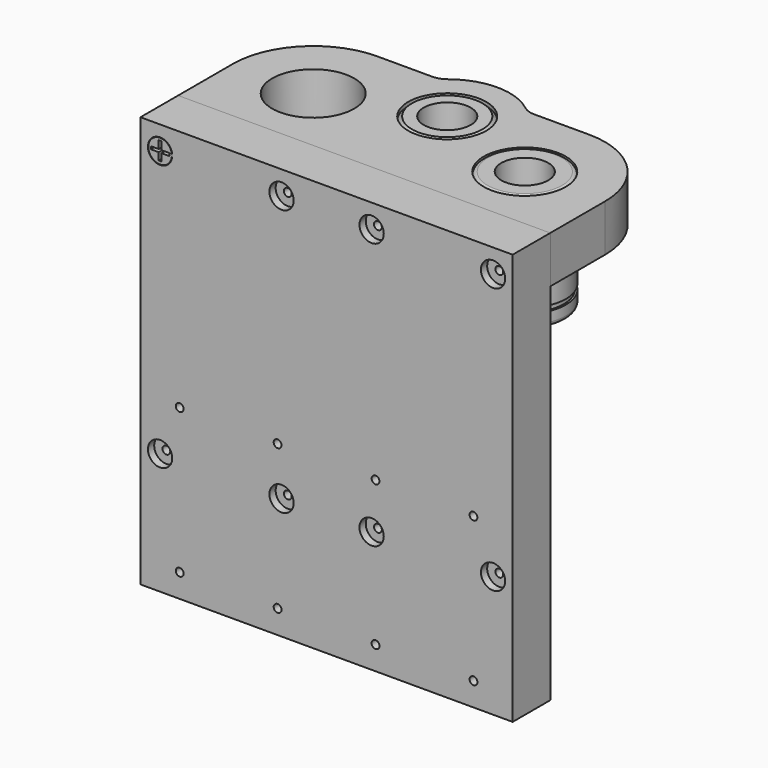
from build123d import *

# Parameters (mm, degrees)
F0_W      = 95
F0_H      = 80
F1_DEPTH  = 12
F2_R      = 10.475
F3_DEPTH  = 12
F4_R      = 9.975
F5_DEPTH  = 25
F6_R      = 10.5
F6_R_2    = 6
F7_DEPTH  = 30
F9_START  = -3.5
F8_R      = 13.9480454754
F8_R_2    = 10
F9_DEPTH  = 1.3
F11_START = -3.5
F10_R     = 14.6955703702
F10_R_2   = 10
F11_DEPTH = 1.3
F12_R     = 1
F13_R     = 1
F14_DEPTH = 25
F15_R     = 3.1
F16_DEPTH = 2
F17_R     = 3
F18_DEPTH = 2
F19_R     = 0.95
F20_DEPTH = 23
F22_DEPTH = 1.5
F23_W     = 95
F23_H     = 25
F24_DEPTH = 12
F25_R     = 1
F26_DEPTH = 25
F27_R     = 3.1
F28_DEPTH = 2
F29_R     = 10
F29_R_2   = 6
F30_DEPTH = 25
F31_SIZE  = 1
F32_R     = 5


with BuildPart() as f1:
    # F0 (on Front) → F1 (new body)
    with BuildSketch(Plane.XZ):
        with Locations((0, 40)):
            Rectangle(F0_W, F0_H)
    extrude(amount=-F1_DEPTH)


with BuildPart() as f3:
    # F2 (on face) → F3 (new body)
    with BuildSketch(Plane.XY.offset(80)):
        with BuildLine():
            Line((-47.5, 12), (47.5, 12))
            Line((47.5, 12), (47.5, 29.5))
            ThreePointArc((47.5, 29.5), (41.4956890143, 43.9956890143), (27, 50))
            Line((27, 50), (11.1242977306, 50))
            ThreePointArc((11.1242977306, 50), (14.7307291688, 44.7454477946), (16, 38.5))
            ThreePointArc((16, 38.5), (-6.2454477946, 23.7692708312), (-11.1242977306, 50))
            Line((-11.1242977306, 50), (-27, 50))
            ThreePointArc((-27, 50), (-41.4956890143, 43.9956890143), (-47.5, 29.5))
            Line((-47.5, 29.5), (-47.5, 12))
        make_face()
        with Locations((-27, 29.5)):
            Circle(F2_R, mode=Mode.SUBTRACT)
        with Locations((27, 29.5)):
            Circle(F2_R, mode=Mode.SUBTRACT)
        with BuildLine():
            ThreePointArc((16, 38.5), (14.7307291688, 44.7454477946), (11.1242977306, 50))
            Line((11.1242977306, 50), (-11.1242977306, 50))
            ThreePointArc((-11.1242977306, 50), (-6.2454477946, 23.7692708312), (16, 38.5))
        make_face()
        with BuildLine():
            Line((-11.1242977306, 50), (11.1242977306, 50))
            ThreePointArc((11.1242977306, 50), (0, 54.5), (-11.1242977306, 50))
        make_face()
    extrude(amount=-F3_DEPTH)

    # F4 (on face) → F5 (cut)
    with BuildSketch(Plane.XY.offset(80)):
        with Locations((0, 38.5)):
            Circle(F4_R)
    extrude(amount=-F5_DEPTH, mode=Mode.SUBTRACT)


with BuildPart() as f7:
    # F6 (on face) → F7 (new body)
    with BuildSketch(Plane.XY.offset(80)):
        with Locations((27, 29.5)):
            Circle(F6_R)
        with Locations((27, 29.5)):
            Circle(F6_R_2, mode=Mode.SUBTRACT)
    extrude(amount=-F7_DEPTH)

    # F8 (on face) → F9 (cut)
    with BuildSketch(Plane.XY.offset(80).offset(F9_START)):
        with Locations((27, 29.5)):
            Circle(F8_R)
        with Locations((27, 29.5)):
            Circle(F8_R_2, mode=Mode.SUBTRACT)
    extrude(amount=-F9_DEPTH, mode=Mode.SUBTRACT)

    # F10 (on face) → F11 (cut)
    with BuildSketch(Plane(origin=(0, 0, 50), x_dir=(1, 0, 0), z_dir=(0, 0, -1)).offset(F11_START)):
        with Locations((27, -29.5)):
            Circle(F10_R)
        with Locations((27, -29.5)):
            Circle(F10_R_2, mode=Mode.SUBTRACT)
    extrude(amount=-F11_DEPTH, mode=Mode.SUBTRACT)

    # F12
    f12_edges = [f7.edges().sort_by_distance(p)[0] for p in [
        (16.5, 29.5, 80),
        (16.5, 29.5, 50),
    ]]
    fillet(f12_edges, radius=F12_R)


with BuildPart() as f14_tool:
    # F13 (on face) → F14 (new body)
    with BuildSketch(Plane.XZ):
        with Locations((-42.5, 74)):
            Circle(F13_R)
        with Locations((-11.5, 74)):
            Circle(F13_R)
        with Locations((11.5, 74)):
            Circle(F13_R)
        with Locations((42.5, 74)):
            Circle(F13_R)
        with Locations((-42.5, 6)):
            Circle(F13_R)
        with Locations((-11.5, 6)):
            Circle(F13_R)
        with Locations((11.5, 6)):
            Circle(F13_R)
        with Locations((42.5, 6)):
            Circle(F13_R)
    extrude(amount=-F14_DEPTH)


with BuildPart() as f1_1:
    add(f1.part)

    # F14: cut by f14_tool
    add(f14_tool.part, mode=Mode.SUBTRACT)

    # F15 (on face) → F16 (cut)
    with BuildSketch(Plane.XZ):
        with Locations((-42.5, 74)):
            Circle(F15_R)
        with Locations((-11.5, 74)):
            Circle(F15_R)
        with Locations((11.5, 74)):
            Circle(F15_R)
        with Locations((42.5, 74)):
            Circle(F15_R)
        with Locations((-42.5, 6)):
            Circle(F15_R)
        with Locations((-11.5, 6)):
            Circle(F15_R)
        with Locations((11.5, 6)):
            Circle(F15_R)
        with Locations((42.5, 6)):
            Circle(F15_R)
    extrude(amount=-F16_DEPTH, mode=Mode.SUBTRACT)

    # F23 (on face) → F24 (join)
    with BuildSketch(Plane.XZ):
        with Locations((0, -12.5)):
            Rectangle(F23_W, F23_H)
    extrude(amount=-F24_DEPTH)

    # F25 (on face) → F26 (cut)
    with BuildSketch(Plane(origin=(0, 12, 0), x_dir=(-1, 0, 0), z_dir=(0, 1, 0))):
        with Locations((-37.5, -19)):
            Circle(F25_R)
        with Locations((-37.5, 18)):
            Circle(F25_R)
        with Locations((-12.5, -19)):
            Circle(F25_R)
        with Locations((-12.5, 18)):
            Circle(F25_R)
        with Locations((12.5, -19)):
            Circle(F25_R)
        with Locations((12.5, 18)):
            Circle(F25_R)
        with Locations((37.5, -19)):
            Circle(F25_R)
        with Locations((37.5, 18)):
            Circle(F25_R)
    extrude(amount=-F26_DEPTH, mode=Mode.SUBTRACT)

    # F27 (on face) → F28 (cut)
    with BuildSketch(Plane(origin=(0, 12, 0), x_dir=(-1, 0, 0), z_dir=(0, 1, 0))):
        with Locations((-37.5, 18)):
            Circle(F27_R)
        with Locations((-37.5, -19)):
            Circle(F27_R)
        with Locations((-12.5, 18)):
            Circle(F27_R)
        with Locations((-12.5, -19)):
            Circle(F27_R)
        with Locations((12.5, 18)):
            Circle(F27_R)
        with Locations((12.5, -19)):
            Circle(F27_R)
        with Locations((37.5, 18)):
            Circle(F27_R)
        with Locations((37.5, -19)):
            Circle(F27_R)
    extrude(amount=-F28_DEPTH, mode=Mode.SUBTRACT)


with BuildPart() as f3_1:
    add(f3.part)

    # F14: cut by f14_tool
    add(f14_tool.part, mode=Mode.SUBTRACT)

    # F32
    f32_edges = [f3_1.edges().sort_by_distance(p)[0] for p in [
        (11.124298, 50, 74),
        (-11.124298, 50, 74),
    ]]
    fillet(f32_edges, radius=F32_R)


with BuildPart() as f18:
    # F17 (on face) → F18 (new body)
    with BuildSketch(Plane.XZ):
        with Locations((-42.5, 74)):
            Circle(F17_R)
    extrude(amount=-F18_DEPTH)

    # F19 (on face) → F20 (join)
    with BuildSketch(Plane(origin=(0, 2, 0), x_dir=(-1, 0, 0), z_dir=(0, 1, 0))):
        with Locations((42.5, 74)):
            Circle(F19_R)
    extrude(amount=F20_DEPTH)

    # F21 (on face) → F22 (cut)
    with BuildSketch(Plane.XZ):
        Polygon((-40.15, 73.65), (-40.15, 74.35), (-42.15, 74.35), (-42.15, 76.35), (-42.85, 76.35), (-42.85, 74.35), (-44.85, 74.35), (-44.85, 73.65), (-42.85, 73.65), (-42.85, 71.7780768571), (-42.15, 71.7780768571), (-42.15, 73.65), align=None)
    extrude(amount=-F22_DEPTH, mode=Mode.SUBTRACT)


with BuildPart() as f30:
    # F29 (on face) → F30 (new body)
    with BuildSketch(Plane.XY.offset(80)):
        with Locations((0, 38.5)):
            Circle(F29_R)
        with Locations((0, 38.5)):
            Circle(F29_R_2, mode=Mode.SUBTRACT)
    extrude(amount=-F30_DEPTH)

    # F31
    f31_edges = [f30.edges().sort_by_distance(p)[0] for p in [
        (-10, 38.5, 55),
        (-10, 38.5, 80),
    ]]
    chamfer(f31_edges, length=F31_SIZE)


solid = Compound([f7.part, f1_1.part, f3_1.part, f18.part, f30.part])
